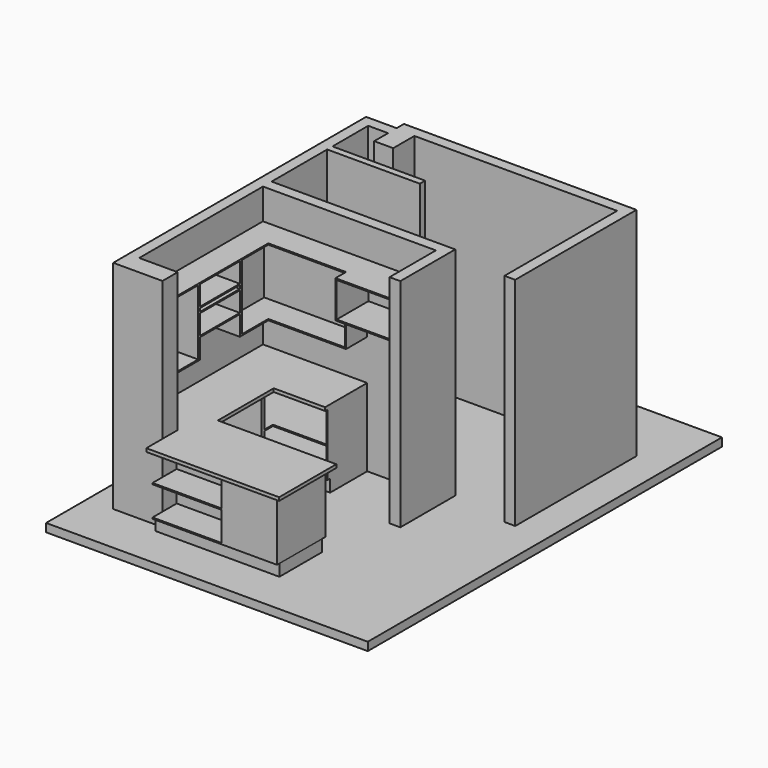
from build123d import *

# Parameters (mm, degrees)
F0_W      = 1120
F0_H      = 80
F1_DEPTH  = 2620
F2_W      = 1260
F2_H      = 820
F2_W_2    = 1230
F2_H_2    = 790
F3_DEPTH  = 320
F5_DEPTH  = 320
F6_DEPTH  = 15
F7_W      = 600
F7_H      = 15
F8_DEPTH  = 320
F9_W      = 505
F9_H      = 820
F9_W_2    = 475
F9_H_2    = 790
F10_DEPTH = 320
F11_DEPTH = 150
F12_W     = 1260
F12_H     = 750
F12_W_2   = 779.1761636734
F12_H_2   = 15
F12_W_3   = 450.8238363266
F13_DEPTH = 600
F14_W     = 50
F14_H     = 720
F14_W_2   = 125
F14_H_2   = 15
F15_DEPTH = 600
F16_W     = 830
F16_H     = 450
F16_W_2   = 800
F16_H_2   = 420
F17_DEPTH = 480
F18_W     = 3888.2797956467
F18_H     = 5350.5387306213
F19_DEPTH = 100
F21_DEPTH = 700
F22_W     = 149.9238204956
F22_H     = 15
F23_DEPTH = 835
F24_W     = 15
F24_H     = 720
F25_DEPTH = 670
F26_W     = 400
F26_H     = 50
F26_W_2   = 15
F26_H_2   = 720
F27_DEPTH = 715
F29_DEPTH = 40
F30_W     = 835
F30_H     = 15
F31_DEPTH = 364.9238204956


# Not quite as in the source:
# - a feature names something its author has since deleted; it is built from what else it names


with BuildPart() as f1:
    # F0 (on Top) → F1 (new body)
    with BuildSketch(Plane.XY):
        Polygon((-2070, 0), (-2070, -130), (-810, -130), (20, -130), (20, -830), (150, -830), (150, 0), align=None)
        Polygon((-1830, 1460), (-1830, 1590), (-2200, 1590), (-2200, -2000), (-2070, -2000), (-2070, -130), (-2070, 0), (-2070, 840), (-2070, 920), (-2070, 1460), align=None)
        Polygon((980, 1700), (-1600, 1700), (-1600, 1570), (850, 1570), (850, -130), (980, -132.1084350348), align=None)
        Polygon((-1600, 1570), (-1600, 1700), (-1830, 1700), (-1830, 1590), (-1830, 1460), (-1830, 1250), (-1600, 1250), align=None)
        Polygon((-2070, -2000), (-2200, -2000), (-2200, -2230), (-1605, -2230), (-1605, -2000), align=None)
        with Locations((-1510, 880)):
            Rectangle(F0_W, F0_H)
    extrude(amount=F1_DEPTH)

    # F2 (on face) → F3 (join)
    with BuildSketch(Plane.XZ.offset(130)):
        with Locations((-1440, 1840)):
            Rectangle(F2_W, F2_H)
        with Locations((-1440, 1840)):
            Rectangle(F2_W_2, F2_H_2, mode=Mode.SUBTRACT)
    extrude(amount=F3_DEPTH)

    # F4 (on face) → F5 (join)
    with BuildSketch(Plane.YZ.offset(-2070)):
        Polygon((-450, 2235), (-450, 2250), (-865, 2250), (-865, 1430), (-450, 1430), (-450, 1445), (-630, 1445), (-645, 1445), (-850, 1445), (-850, 2235), (-645, 2235), (-630, 2235), align=None)
    extrude(amount=F5_DEPTH)

    # F6 (add): a face of the model
    f6_faces = [f1.faces().sort_by_distance(p)[0] for p in [
        (-2070, -650, 1840),
    ]]
    extrude(f6_faces, amount=F6_DEPTH)

    # F7 (on face) → F8 (join)
    with BuildSketch(Plane.YZ.offset(-2070)):
        Polygon((-865, 1430), (-865, 2250), (-1495, 2250), (-1495, 1430), (-1480, 1430), (-1480, 1670), (-1480, 1685), (-1480, 1925), (-1480, 1940), (-1480, 1980), (-1480, 1995), (-1480, 2235), (-880, 2235), (-880, 1995), (-880, 1980), (-880, 1940), (-880, 1925), (-880, 1685), (-880, 1670), (-880, 1430), align=None)
        with Locations((-1180, 1987.5)):
            Rectangle(F7_W, F7_H)
        with Locations((-1180, 1932.5)):
            Rectangle(F7_W, F7_H)
        with Locations((-1180, 1677.5)):
            Rectangle(F7_W, F7_H)
    extrude(amount=F8_DEPTH)

    # F9 (on face) → F10 (join)
    with BuildSketch(Plane.YZ.offset(-2070)):
        with Locations((-1747.5, 1840)):
            Rectangle(F9_W, F9_H)
        with Locations((-1747.5, 1840)):
            Rectangle(F9_W_2, F9_H_2, mode=Mode.SUBTRACT)
    extrude(amount=F10_DEPTH)

    # F0 (on Top) → F11 (join)
    with BuildSketch(Plane.XY):
        Polygon((-2070, -130), (-2070, -2000), (-1605, -2000), (-1605, -2230), (-1605, -2332), (-110, -2332), (-110, -1690), (-1510, -1690), (-1510, -690), (-810, -690), (-810, -130), align=None)
    extrude(amount=F11_DEPTH)

    # F12 (on face) → F13 (join)
    with BuildSketch(Plane.XZ.offset(130)):
        with Locations((-1440, 525)):
            Rectangle(F12_W, F12_H)
        Polygon((-825, 510), (-825, 165), (-2055, 165), (-2055, 510), (-2055, 525), (-2055, 885), (-825, 885), (-825, 525), align=None, mode=Mode.SUBTRACT)
        with Locations((-1214.5880818367, 517.5)):
            Rectangle(F12_W_2, F12_H_2)
        with Locations((-1829.5880818367, 517.5)):
            Rectangle(F12_W_3, F12_H_2)
    extrude(amount=F13_DEPTH)

    # F14 (on face) → F15 (join)
    with BuildSketch(Plane.YZ.offset(-2070)):
        with Locations((-1500, 525)):
            Rectangle(F14_W, F14_H)
        Polygon((-905, 885), (-905, 165), (-855, 165), (-855, 510), (-855, 525), (-855, 885), align=None)
        with Locations((-792.5, 517.5)):
            Rectangle(F14_W_2, F14_H_2)
        Polygon((-1475, 165), (-1525, 165), (-1985, 165), (-1985, 885), (-1525, 885), (-1475, 885), (-905, 885), (-855, 885), (-730, 885), (-730, 900), (-2000, 900), (-2000, 150), (-730, 150), (-730, 165), (-855, 165), (-905, 165), align=None)
    extrude(amount=F15_DEPTH)

    # F16 (on face) → F17 (join)
    with BuildSketch(Plane.XZ.offset(130)):
        with Locations((-395, 2025)):
            Rectangle(F16_W, F16_H)
        with Locations((-395, 2025)):
            Rectangle(F16_W_2, F16_H_2, mode=Mode.SUBTRACT)
    extrude(amount=F17_DEPTH)

    # F20 (on face) → F21 (join)
    with BuildSketch(Plane.YZ.offset(-1470)):
        Polygon((-1690, 150), (-1650, 150), (-1650, 165), (-1985, 165), (-1985, 885), (-1650, 885), (-1650, 900), (-2000, 900), (-2000, 150), align=None)
    extrude(amount=F21_DEPTH)

    # F22 (on face) → F23 (join)
    with BuildSketch(Plane.YZ.offset(-1605)):
        Polygon((-2230, 165), (-2230, 150), (-2000, 150), (-2000, 900), (-2230, 900), (-2230, 885), (-2015, 885), (-2015, 165), align=None)
        with Locations((-2304.9619102478, 892.5)):
            Rectangle(F22_W, F22_H)
        with Locations((-2304.9619102478, 157.5)):
            Rectangle(F22_W, F22_H)
    extrude(amount=F23_DEPTH)

    # F24 (on face) → F25 (join)
    with BuildSketch(Plane.YZ.offset(-770)):
        with Locations((-2372.4238204956, 525)):
            Rectangle(F24_W, F24_H)
        Polygon((-1690, 150), (-1650, 150), (-1650, 165), (-1985, 165), (-2015, 165), (-2364.9238204956, 165), (-2379.9238204956, 165), (-2379.9238204956, 150), (-2332, 150), align=None)
        Polygon((-2015, 885), (-1985, 885), (-1650, 885), (-1650, 900), (-2379.9238204956, 900), (-2379.9238204956, 885), (-2364.9238204956, 885), align=None)
    extrude(amount=F25_DEPTH)

    # F26 (on face) → F27 (join)
    with BuildSketch(Plane(origin=(0, -2364.9238204956, 0), x_dir=(-1, 0, 0), z_dir=(0, 1, 0))):
        Polygon((515, 295), (515, 165), (530, 165), (530, 885), (515, 885), (515, 835), (515, 705), (515, 655), (515, 525), (515, 475), (515, 345), align=None)
        with Locations((315, 860)):
            Rectangle(F26_W, F26_H)
        with Locations((315, 680)):
            Rectangle(F26_W, F26_H)
        with Locations((315, 500)):
            Rectangle(F26_W, F26_H)
        with Locations((762.5, 525)):
            Rectangle(F26_W_2, F26_H_2)
        with Locations((315, 320)):
            Rectangle(F26_W, F26_H)
        Polygon((100, 885), (100, 165), (115, 165), (115, 295), (115, 345), (115, 475), (115, 525), (115, 655), (115, 705), (115, 835), (115, 885), align=None)
    extrude(amount=F27_DEPTH)

    # F28 (on face) → F29 (join)
    with BuildSketch(Plane.XY.offset(900)):
        Polygon((-2070, -2000), (-1605, -2000), (-1605, -2230), (-1605, -2379.9238204956), (-100, -2379.9238204956), (-100, -1650), (-1470, -1650), (-1470, -730), (-810, -730), (-810, -130), (-2070, -130), align=None)
        Polygon((-100, -2379.9238204956), (-1605, -2379.9238204956), (-1605, -2473.8321304321), (0, -2473.8321304321), (0, -1609.8160743713), (-1431.3893318176, -1609.8160743713), (-1431.3893318176, -766.4950489998), (-810, -766.4950489998), (-810, -730), (-1470, -730), (-1470, -1650), (-100, -1650), align=None)
    extrude(amount=F29_DEPTH)

    # F30 (on face) → F31 (join, through all)
    with BuildSketch(Plane.XZ.offset(2015)):
        with Locations((-1187.5, 524.5)):
            Rectangle(F30_W, F30_H)
    extrude(amount=F31_DEPTH)


with BuildPart() as f19:
    # F18 (on face) → F19 (new body)
    with BuildSketch(Plane(origin=(0, 0, 0), x_dir=(1, 0, 0), z_dir=(0, 0, -1))):
        with Locations((-573.2000470161, 172.4932193756)):
            Rectangle(F18_W, F18_H)
        Polygon((-810, 130), (20, 130), (20, 830), (150, 830), (150, 0), (-2070, 0), (-2070, -840), (-950, -840), (-950, -920), (-2070, -920), (-2070, -1460), (-1830, -1460), (-1830, -1250), (-1600, -1250), (-1600, -1570), (850, -1570), (850, 130), (980, 132.1084350348), (980, -1700), (-1830, -1700), (-1830, -1590), (-2200, -1590), (-2200, 2230), (-1605, 2230), (-1605, 2332), (-110, 2332), (-110, 1690), (-1510, 1690), (-1510, 690), (-810, 690), align=None, mode=Mode.SUBTRACT)
    extrude(amount=F19_DEPTH)


solid = Compound([f1.part, f19.part])
